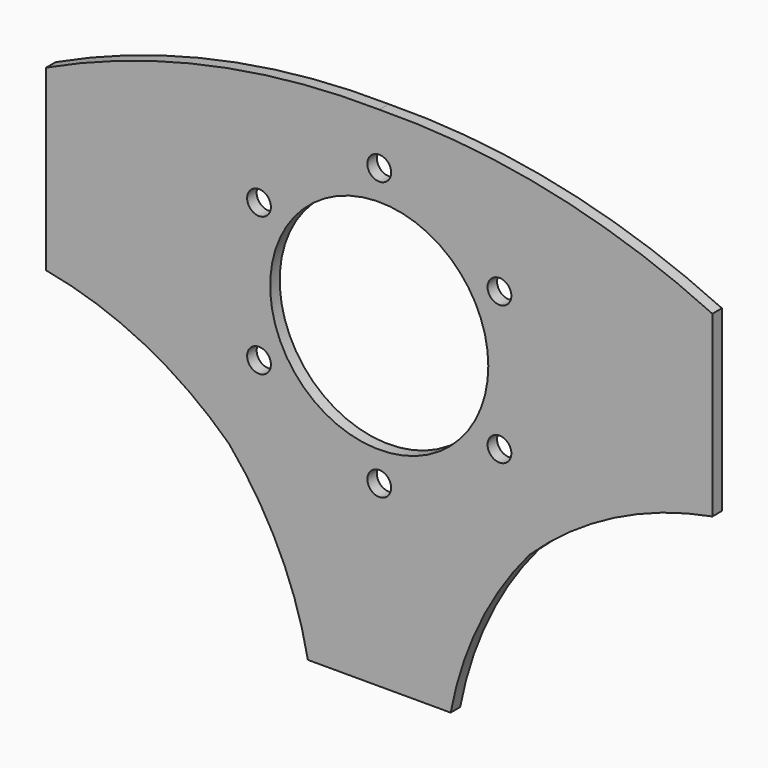
from build123d import *

# Parameters (mm, degrees)
F0_R     = 3
F1_DEPTH = 3


# Not quite as in the source:
# - a feature names something its author has since deleted; it is built from what else it names


with BuildPart() as f1:
    # F0 (on Front) → F1 (new body)
    with BuildSketch(Plane.XZ):
        with BuildLine():
            ThreePointArc((18, -80), (25.2450835608, -57.9435000854), (37.8911830779, -38.474124356))
            ThreePointArc((37.8911830779, -38.474124356), (59.2223421632, -23.3521866114), (84, -15))
            Line((84, -15), (84, 30))
            ThreePointArc((84, 30), (43.0306603199, 43.8097481595), (0, 48))
            ThreePointArc((0, 48), (-43.0306603199, 43.8097481595), (-84, 30))
            Line((-84, 30), (-84, -15))
            ThreePointArc((-84, -15), (-59.2223421632, -23.3521866114), (-37.8911830779, -38.474124356))
            ThreePointArc((-37.8911830779, -38.474124356), (-25.2450835608, -57.9435000854), (-18, -80))
            Line((-18, -80), (0, -80))
            Line((0, -80), (18, -80))
        make_face()
        with Locations((-30.3108891325, -17.5)):
            Circle(F0_R, mode=Mode.SUBTRACT)
        with Locations((0, -35)):
            Circle(F0_R, mode=Mode.SUBTRACT)
        with Locations((30.3108891325, -17.5)):
            Circle(F0_R, mode=Mode.SUBTRACT)
        with Locations((-30.3108891325, 17.5)):
            Circle(F0_R, mode=Mode.SUBTRACT)
        with BuildLine():
            ThreePointArc((19.2964358267, -19.5933040702), (-25.3663358138, 10.6206877076), (27.5, 0))
            ThreePointArc((27.5, 0), (25.3663358138, -10.6206877076), (19.2964358267, -19.5933040702))
        make_face(mode=Mode.SUBTRACT)
        with Locations((30.3108891325, 17.5)):
            Circle(F0_R, mode=Mode.SUBTRACT)
        with Locations((0, 35)):
            Circle(F0_R, mode=Mode.SUBTRACT)
    extrude(amount=F1_DEPTH)


solid = f1.part
